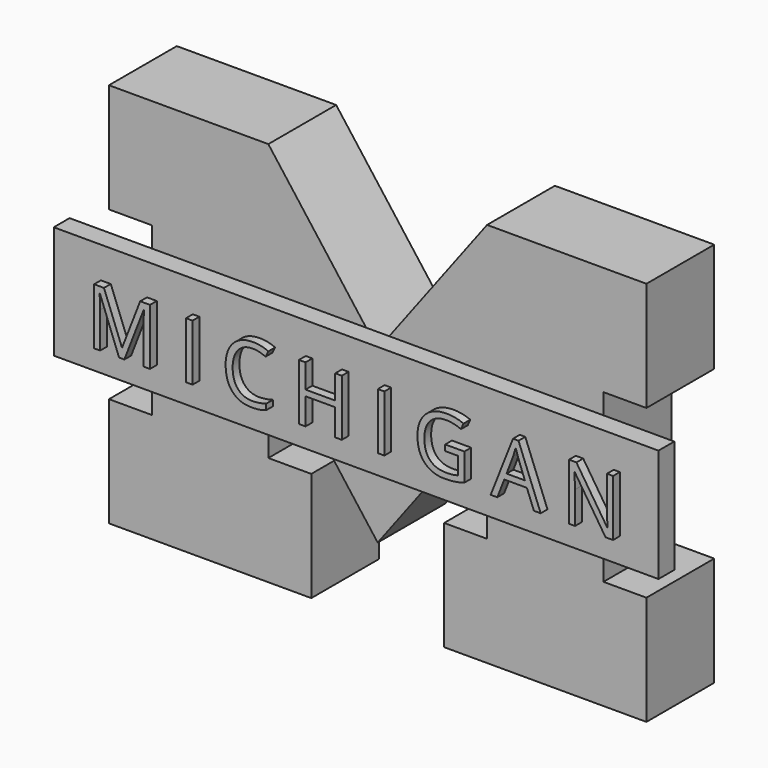
from build123d import *

# Parameters (mm, degrees)
F1_DEPTH     = 7.62
F2_W         = 54.356
F2_H         = 10.16
F3_DEPTH     = 1.778
F4_TEXT_SIZE = 7.1036873685
F5_DEPTH     = 0.762


# Not quite as in the source:
# - Text() gives the source's letters only with a copy of the font that has no kerning and outlines rounded to 1/6400 em; it was checked with that copy


with BuildPart() as f1:
    # F0 (on Front) → F1 (new body)
    with BuildSketch(Plane.XZ):
        Polygon((0, 9.8298), (0, 0), (18.1864, 0), (18.1864, 9.8298), (14.3256, 9.8298), (14.3256, 19.3802), (24.1554, 6.3356148124), (33.9852, 19.3802), (33.9852, 9.8298), (30.1244, 9.8298), (30.1244, 0), (48.3108, 0), (48.3108, 9.8298), (44.45, 9.8298), (44.45, 24.8412), (48.3108, 24.8412), (48.3108, 34.671), (33.9852, 34.671), (24.1554, 21.6264148124), (14.3256, 34.671), (0, 34.671), (0, 24.8412), (3.8608, 24.8412), (3.8608, 9.8298), align=None)
    extrude(amount=F1_DEPTH)

    # F2 (on face) → F3 (join)
    with BuildSketch(Plane.XZ.offset(7.62)):
        with Locations((23.6379163055, 17.9242822024)):
            Rectangle(F2_W, F2_H)
    extrude(amount=F3_DEPTH)

    # F4 (on face) → F5 (join)
    with BuildSketch(Plane.XZ.offset(9.398)):
        with Locations((0, 15.1103549084)):
            Text('M I C H I G A N', F4_TEXT_SIZE, font='Open Sans', text_align=(TextAlign.LEFT, TextAlign.BOTTOM))
    extrude(amount=F5_DEPTH)


solid = f1.part
